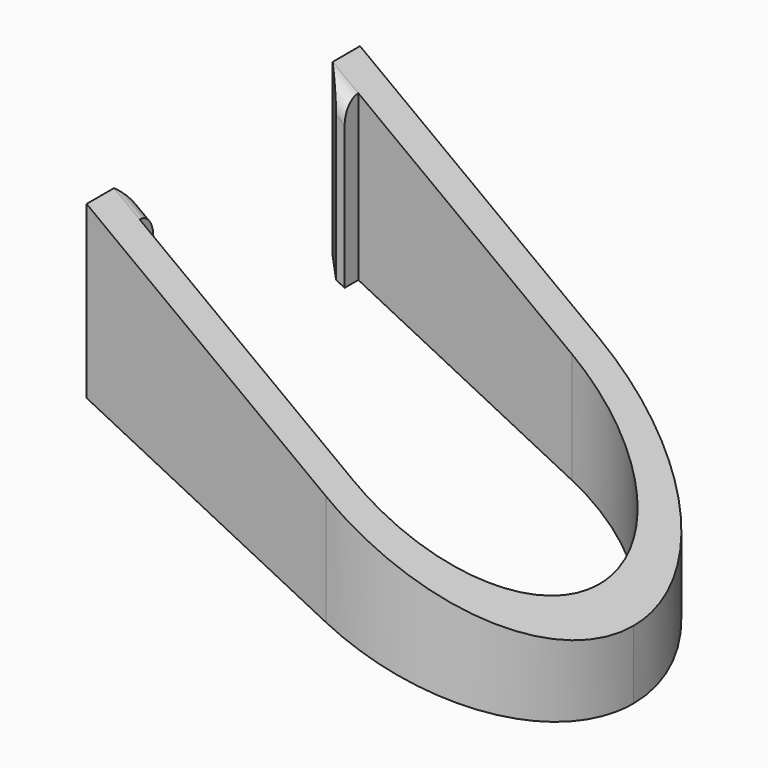
from build123d import *

# Parameters (mm, degrees)
F1_DEPTH    = 34.925
F3_DEPTH    = 31.75
F4_T1_DEPTH = 8.9296875
F4_T3_DEPTH = 8.9296875


# Not quite as in the source:
# - a fillet or chamfer that OpenCascade refuses, or shapes differently, is made with other operations: its cross-section is extruded or revolved along the edge and cut away or added


with BuildPart() as f1:
    # F0 (on Top) → F1 (new body)
    with BuildSketch(Plane.XY):
        with BuildLine():
            Line((0, 15.875), (-22.225, 15.875))
            Line((-22.225, 15.875), (-22.225, 12.7))
            Line((-22.225, 12.7), (-20.6375, 11.1125))
            Line((-20.6375, 11.1125), (-19.84375, 11.1125))
            Line((-19.84375, 11.1125), (-19.84375, 12.7))
            Line((-19.84375, 12.7), (0, 12.7))
            ThreePointArc((0, 12.7), (8.9802561211, 8.9802561211), (12.7, 0))
            ThreePointArc((12.7, 0), (8.9802561211, -8.9802561211), (0, -12.7))
            Line((0, -12.7), (-19.84375, -12.7))
            Line((-19.84375, -12.7), (-19.84375, -11.1125))
            Line((-19.84375, -11.1125), (-20.6375, -11.1125))
            Line((-20.6375, -11.1125), (-22.225, -12.7))
            Line((-22.225, -12.7), (-22.225, -15.875))
            Line((-22.225, -15.875), (0, -15.875))
            ThreePointArc((0, -15.875), (11.2253201513, -11.2253201513), (15.875, 0))
            ThreePointArc((15.875, 0), (11.2253201513, 11.2253201513), (0, 15.875))
        make_face()
    extrude(amount=F1_DEPTH)

    # F2 (on face) → F3 (cut, through all)
    with BuildSketch(Plane.XZ.offset(15.875)):
        Polygon((0, 18.25625), (0, 34.925), (-22.225, 34.925), align=None)
        Polygon((15.875, 6.35), (15.875, 34.925), (0, 34.925), (0, 18.25625), align=None)
        Polygon((-22.225, 0), (0, 0), (0, 7.9375), (-22.225, 19.05), align=None)
        Polygon((0, 0), (15.875, 0), (0, 7.9375), align=None)
    extrude(amount=-F3_DEPTH, mode=Mode.SUBTRACT)

    # F4: fillet of radius 1.5875 on 2 edges, made by hand

    # F4_s2 → F4_t1 (cut)
    with BuildSketch(Plane(origin=(-25.43175, 0, 19.0738125), x_dir=(0, 1, 0), z_dir=(-0.8, 0, 0.6))):
        with BuildLine():
            ThreePointArc((12.7, -14.605), (11.5774679849, -14.1400320151), (11.1125, -13.0175))
            Line((11.1125, -13.0175), (11.1125, -14.605))
            Line((11.1125, -14.605), (12.7, -14.605))
        make_face()
    extrude(amount=F4_T1_DEPTH, mode=Mode.SUBTRACT)

    # F4_s4 → F4_t3 (cut)
    with BuildSketch(Plane(origin=(-32.5755, 0, 24.431625), x_dir=(0, 1, 0), z_dir=(0.8, 0, -0.6))):
        with BuildLine():
            ThreePointArc((-12.7, 14.605), (-11.5774679849, 14.1400320151), (-11.1125, 13.0175))
            Line((-11.1125, 13.0175), (-11.1125, 14.605))
            Line((-11.1125, 14.605), (-12.7, 14.605))
        make_face()
    extrude(amount=F4_T3_DEPTH, mode=Mode.SUBTRACT)


solid = f1.part
